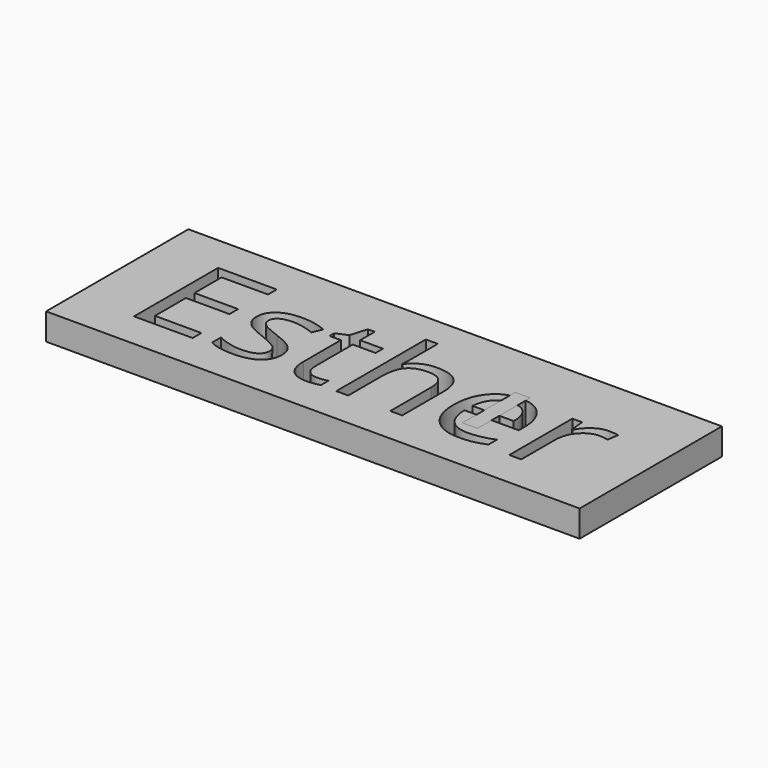
from build123d import *

# Parameters (mm, degrees)
F0_W         = 152.4
F0_H         = 50.8
F1_DEPTH     = 7.62
F2_TEXT_SIZE = 42.0551559994
F3_DEPTH     = 113.792
F4_W         = 4.2979175045
F4_H         = 5.0218522942
F5_DEPTH     = 7.62


# Not quite as in the source:
# - Text() gives the source's letters only with a copy of the font that has no kerning and outlines rounded to 1/6400 em; it was checked with that copy


with BuildPart() as f1:
    # F0 (on Top) → F1 (new body)
    with BuildSketch(Plane.XY):
        Rectangle(F0_W, F0_H)
    extrude(amount=F1_DEPTH)

    # F2 (on Top) → F3 (cut)
    with BuildSketch(Plane.XY):
        with Locations((-63.5, -15.0397123196)):
            Text('Esther', F2_TEXT_SIZE, font='Open Sans', text_align=(TextAlign.LEFT, TextAlign.BOTTOM))
    extrude(amount=F3_DEPTH, mode=Mode.SUBTRACT)


with BuildPart() as f5:
    # F4 (on face) → F5 (new body)
    with BuildSketch(Plane.XY.offset(7.62)):
        with BuildLine():
            Line((29.9507501625, -4.4010720753), (34.248667667, -4.4010720753))
            Line((34.248667667, -4.4010720753), (34.248667667, 7.7978295579))
            add(Edge.make_bspline(
                [(29.9507501625, 7.500612047), (30.0751887604, 7.5359171672), (30.2002089046, 7.5692059584), (30.3257646897, 7.6004958365), (30.4518116035, 7.6298074292), (30.5783066221, 7.6571641753), (30.7052083035, 7.6825919241), (30.8324768816, 7.7061185347), (31.1910598589, 7.766974699), (31.4231211509, 7.8000417557), (31.6560367409, 7.82715134), (31.8896044877, 7.8484957802), (32.1236421179, 7.8642780057), (32.3579877383, 7.8747065149), (32.5925003486, 7.8799903422), (32.8949371139, 7.8804334801), (32.9628138902, 7.8801221802), (33.0306843623, 7.8793964016), (33.098544688, 7.8782510812), (33.1663923859, 7.8766803742), (33.2342252178, 7.8746782107), (33.3020400706, 7.8722388527), (33.4800133742, 7.8646743265), (33.5901352356, 7.8588227147), (33.7001821236, 7.8517787054), (33.8101374547, 7.8435181828), (33.9199833803, 7.8340169701), (34.0297008062, 7.8232509748), (34.1392694114, 7.8111963337), (34.248667667, 7.7978295579)],
                knots=[0.6875770325, 0.6875770325, 0.6875770325, 0.6875770325, 0.6875770325, 0.6875770325, 0.6875770325, 0.6875770325, 0.6875770325, 0.7053227635, 0.7053227635, 0.7053227635, 0.7053227635, 0.7053227635, 0.7053227635, 0.7053227635, 0.7374472737, 0.7374472737, 0.7374472737, 0.7374472737, 0.7374472737, 0.7374472737, 0.7374472737, 0.746743435, 0.746743435, 0.746743435, 0.746743435, 0.746743435, 0.746743435, 0.746743435, 0.7618524276, 0.7618524276, 0.7618524276, 0.7618524276, 0.7618524276, 0.7618524276, 0.7618524276, 0.7618524276, 0.7618524276], degree=8))
            Line((29.9507501625, 7.500612047), (29.9507501625, -4.4010720753))
        make_face()
        with BuildLine():
            add(Edge.make_bspline(
                [(29.9507501625, 7.500612047), (30.0751887604, 7.5359171672), (30.2002089046, 7.5692059584), (30.3257646897, 7.6004958365), (30.4518116035, 7.6298074292), (30.5783066221, 7.6571641753), (30.7052083035, 7.6825919241), (30.8324768816, 7.7061185347), (31.1910598589, 7.766974699), (31.4231211509, 7.8000417557), (31.6560367409, 7.82715134), (31.8896044877, 7.8484957802), (32.1236421179, 7.8642780057), (32.3579877383, 7.8747065149), (32.5925003486, 7.8799903422), (32.8949371139, 7.8804334801), (32.9628138902, 7.8801221802), (33.0306843623, 7.8793964016), (33.098544688, 7.8782510812), (33.1663923859, 7.8766803742), (33.2342252178, 7.8746782107), (33.3020400706, 7.8722388527), (33.4800133742, 7.8646743265), (33.5901352356, 7.8588227147), (33.7001821236, 7.8517787054), (33.8101374547, 7.8435181828), (33.9199833803, 7.8340169701), (34.0297008062, 7.8232509748), (34.1392694114, 7.8111963337), (34.248667667, 7.7978295579)],
                knots=[0.6875770325, 0.6875770325, 0.6875770325, 0.6875770325, 0.6875770325, 0.6875770325, 0.6875770325, 0.6875770325, 0.6875770325, 0.7053227635, 0.7053227635, 0.7053227635, 0.7053227635, 0.7053227635, 0.7053227635, 0.7053227635, 0.7374472737, 0.7374472737, 0.7374472737, 0.7374472737, 0.7374472737, 0.7374472737, 0.7374472737, 0.746743435, 0.746743435, 0.746743435, 0.746743435, 0.746743435, 0.746743435, 0.746743435, 0.7618524276, 0.7618524276, 0.7618524276, 0.7618524276, 0.7618524276, 0.7618524276, 0.7618524276, 0.7618524276, 0.7618524276], degree=8))
            Line((34.248667667, 7.7978295579), (34.248667667, 9.4229243696))
            Line((34.248667667, 9.4229243696), (29.9507501625, 9.4229243696))
            Line((29.9507501625, 9.4229243696), (29.9507501625, 7.500612047))
        make_face()
        with Locations((32.0997089148, -6.9119982225)):
            Rectangle(F4_W, F4_H)
    extrude(amount=-F5_DEPTH)


solid = Compound([f1.part, f5.part])
